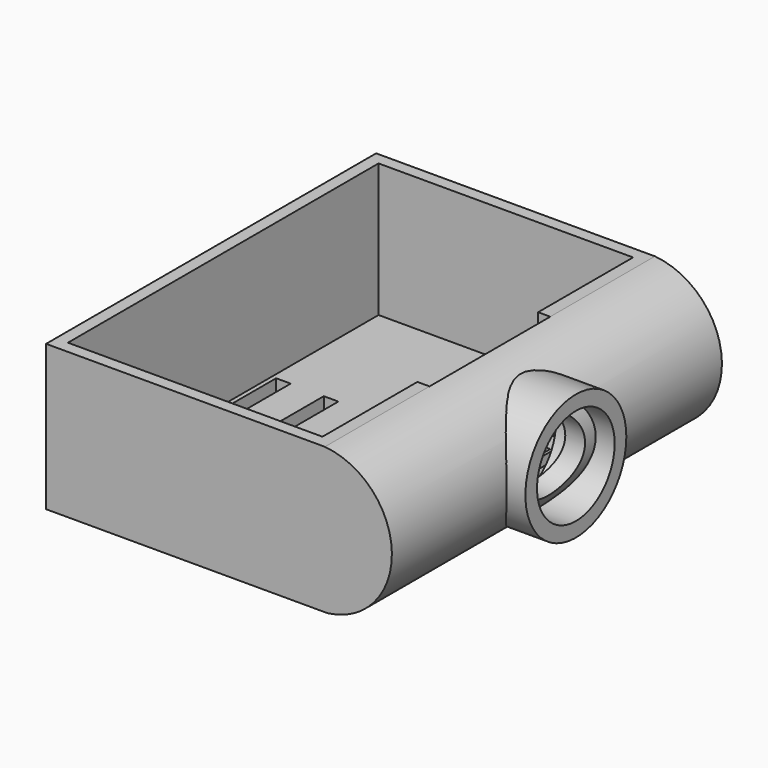
from build123d import *

# Parameters (mm, degrees)
F1_DEPTH  = 42.5
F2_R      = 7.25
F3_DEPTH  = 38.7487115805
F4_W      = 3
F4_H      = 25.0110699423
F4_W_2    = 2.9971426107
F4_H_2    = 25
F5_DEPTH  = 30.0010001
F7_W      = 52.4388903172
F7_H      = 80
F7_W_2    = 2.9971426107
F7_H_2    = 25
F7_W_3    = 3
F7_H_3    = 25.0110699423
F8_DEPTH  = 27.5
F10_DEPTH = 37.5
F11_W     = 73
F11_H     = 20.5
F12_DEPTH = 8
F13_W     = 2.5983742954
F13_H     = 31.0936123133
F14_DEPTH = 26.81786
F16_START = 60.56282
F15_R     = 13
F15_R_2   = 10
F16_DEPTH = 12.08773


# Not quite as in the source:
# - a feature names something its author has since deleted; it is built from what else it names


with BuildPart() as f1:
    # F0 (on Front) → F1 (new body, symmetric)
    with BuildSketch(Plane.XZ):
        with BuildLine():
            Line((-32.5, -15), (25.4704337567, -15))
            ThreePointArc((25.4704337567, -15), (38.745344936, 0.2399153721), (24.9388903172, 15))
            Line((24.9388903172, 15), (22.3945248872, 15))
            Line((22.3945248872, 15), (-32.5, 15))
            Line((-32.5, 15), (-32.5, -15))
        make_face()
        with BuildLine():
            Line((25.399065212, -10.9720011933), (25.0102588618, 10.9720011933))
            ThreePointArc((25.0102588618, 10.9720011933), (34.7459726513, 0.1690540354), (25.399065212, -10.9720011933))
        make_face(mode=Mode.SUBTRACT)
        with BuildLine():
            ThreePointArc((25.399065212, -10.9720011933), (34.7459726513, 0.1690540354), (25.0102588618, 10.9720011933))
            Line((25.0102588618, 10.9720011933), (25.399065212, -10.9720011933))
        make_face()
    extrude(amount=F1_DEPTH, both=True)

    # F2 (on Right) → F3 (cut, through all)
    with BuildSketch(Plane.YZ):
        Circle(F2_R)
    extrude(amount=F3_DEPTH, mode=Mode.SUBTRACT)

    # F4 (on face) → F5 (cut, through all)
    with BuildSketch(Plane(origin=(0, 0, -15), x_dir=(1, 0, 0), z_dir=(0, 0, -1))):
        with Locations((-27.6051664799, 0)):
            Rectangle(F4_W, F4_H)
        with Locations((-17.7152827382, 0.0821705908)):
            Rectangle(F4_W_2, F4_H_2)
        with Locations((-8.9320717379, 0.0786611254)):
            Rectangle(F4_W, F4_H_2)
        with Locations((0.1306068152, -0.1937846464)):
            Rectangle(F4_W, F4_H_2)
    extrude(amount=-F5_DEPTH, mode=Mode.SUBTRACT)

    # F7 (on face) → F8 (cut)
    with BuildSketch(Plane.XY.offset(15)):
        with Locations((-3.7805548414, 0)):
            Rectangle(F7_W, F7_H)
        with Locations((-17.7152827382, -0.0821705908)):
            Rectangle(F7_W_2, F7_H_2, mode=Mode.SUBTRACT)
        with Locations((-8.9320717379, -0.0786611254)):
            Rectangle(F7_W_3, F7_H_2, mode=Mode.SUBTRACT)
        with Locations((-27.6051664799, 0)):
            Rectangle(F7_W_3, F7_H_3, mode=Mode.SUBTRACT)
        with Locations((0.1306068152, 0.1937846464)):
            Rectangle(F7_W_3, F7_H_2, mode=Mode.SUBTRACT)
    extrude(amount=-F8_DEPTH, mode=Mode.SUBTRACT)

    # F9 (on Front) → F10 (cut, symmetric)
    with BuildSketch(Plane.XZ):
        with BuildLine():
            Line((24.8281303793, 11.0828392208), (25.6202220917, -10.8693931252))
            ThreePointArc((25.6202220917, -10.8693931252), (34.6667124862, 0.4474334863), (24.8281303793, 11.0828392208))
        make_face()
    extrude(amount=F10_DEPTH, both=True, mode=Mode.SUBTRACT)

    # F11 (on face) → F12 (cut)
    with BuildSketch(Plane(origin=(22.4388903172, 0, 0), x_dir=(0, -1, 0), z_dir=(-1, 0, 0))):
        with Locations((0, 1.25)):
            Rectangle(F11_W, F11_H)
    extrude(amount=-F12_DEPTH, mode=Mode.SUBTRACT)

    # F13 (on face) → F14 (cut)
    with BuildSketch(Plane.XY.offset(15)):
        with Locations((23.6397031695, 0)):
            Rectangle(F13_W, F13_H)
    extrude(amount=-F14_DEPTH, mode=Mode.SUBTRACT)


with BuildPart() as f16:
    # F15 (on face) → F16 (new body)
    with BuildSketch(Plane.YZ.offset(-30).offset(F16_START)):
        Circle(F15_R)
        Circle(F15_R_2, mode=Mode.SUBTRACT)
    extrude(amount=F16_DEPTH)


solid = Compound([f1.part, f16.part])
